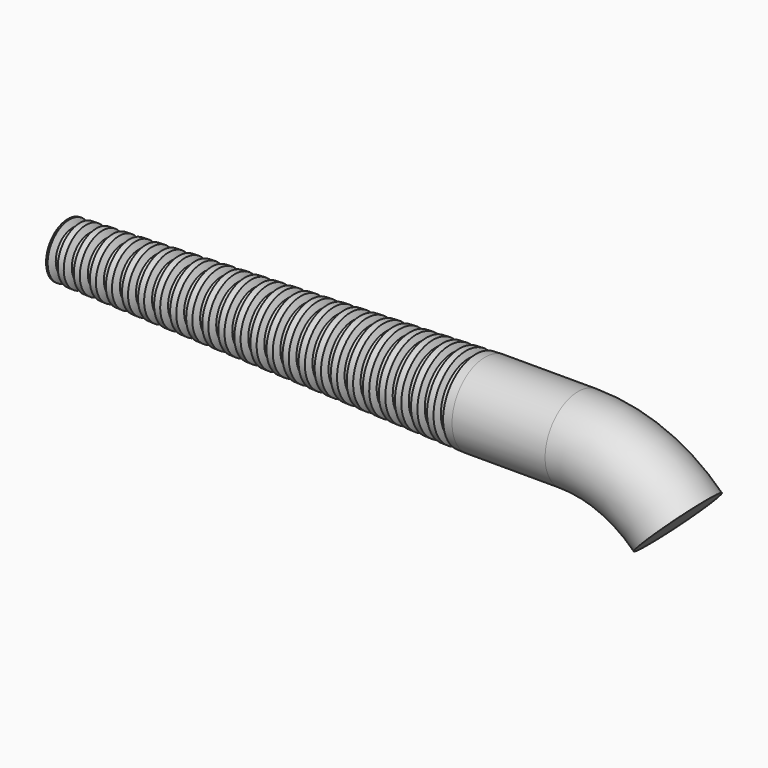
from build123d import *

# Parameters (mm, degrees)
F3_R      = 75
F8_R      = 49.537672475
F13_DEPTH = 232


with BuildPart() as f4:
    # F4: sweep along a path in F0
    with BuildLine(Plane.XZ) as f4_path:
        Line((-350, 75), (-181.066017178, 75))
        ThreePointArc((-181.066017178, 75), (0, 0), (75, -181.066017178))
        Line((75, -181.066017178), (75, -350))
    # F3 (on plane+point) → F4 (sweep)
    with BuildSketch(Plane.YZ.offset(-350)):
        with Locations((0, 75)):
            Circle(F3_R)
    sweep(path=f4_path.line)

    # F8 (on plane+point) → F9 section 0
    with BuildSketch(Plane.YZ.offset(-1107.697725296)):
        with Locations((0, 75)):
            Circle(F8_R)
    # F3 (on plane+point) → F9 section 1
    with BuildSketch(Plane.YZ.offset(-350)):
        with Locations((0, 75)):
            Circle(F3_R)
    loft()

    # F10 (on Front) → F11 (revolve, cut)
    with BuildSketch(Plane.XZ):
        Polygon((-1085.869221311, 125.2712163399), (-1104.697725296, 124.6384870611), (-1099.2664424752, 113.0726968058), (-1090.5117942881, 113.3668955503), align=None)
        Polygon((-1060.530301493, 114.4205035296), (-1055.8877285158, 126.3248243192), (-1074.7162325009, 125.6920950404), (-1069.28494968, 114.1263047851), align=None)
        Polygon((-1030.5488086978, 115.4741115089), (-1025.9062357207, 127.3784322985), (-1044.7347397057, 126.7457030197), (-1039.3034568849, 115.1799127644), align=None)
        Polygon((-1000.5673159027, 116.5277194882), (-995.9247429255, 128.4320402778), (-1014.7532469106, 127.799310999), (-1009.3219640897, 116.2335207437), align=None)
        Polygon((-970.5858231075, 117.5813274675), (-965.9432501303, 129.4856482571), (-984.7717541154, 128.8529189783), (-979.3404712946, 117.287128723), align=None)
        Polygon((-940.6043303123, 118.6349354468), (-935.9617573352, 130.5392562364), (-954.7902613202, 129.9065269576), (-949.3589784994, 118.3407367023), align=None)
        Polygon((-910.6228375172, 119.6885434262), (-905.98026454, 131.5928642158), (-924.8087685251, 130.960134937), (-919.3774857043, 119.3943446816), align=None)
        Polygon((-880.641344722, 120.7421514055), (-875.9987717449, 132.6464721951), (-894.8272757299, 132.0137429163), (-889.3959929091, 120.447952661), align=None)
        Polygon((-850.6598519269, 121.7957593848), (-846.0172789497, 133.7000801744), (-864.8457829348, 133.0673508956), (-859.4145001139, 121.5015606403), align=None)
        Polygon((-820.6783591317, 122.8493673641), (-816.0357861546, 134.7536881537), (-834.8642901396, 134.1209588749), (-829.4330073188, 122.5551686196), align=None)
        Polygon((-790.6968663366, 123.9029753434), (-786.0542933594, 135.807296133), (-804.8827973445, 135.1745668542), (-799.4515145236, 123.6087765989), align=None)
        Polygon((-760.7153735414, 124.9565833227), (-756.0728005643, 136.8609041123), (-774.9013045493, 136.2281748335), (-769.4700217285, 124.6623845782), align=None)
        Polygon((-730.7338807463, 126.010191302), (-726.0913077691, 137.9145120916), (-744.9198117542, 137.2817828128), (-739.4885289333, 125.7159925575), align=None)
        Polygon((-700.7523879511, 127.0637992813), (-696.1098149739, 138.9681200709), (-714.938318959, 138.3353907921), (-709.5070361382, 126.7696005368), align=None)
        Polygon((-670.770895156, 128.1174072606), (-666.1283221788, 140.0217280502), (-684.9568261639, 139.3889987714), (-679.525543343, 127.8232085161), align=None)
        Polygon((-640.7894023608, 129.17101524), (-636.1468293836, 141.0753360296), (-654.9753333687, 140.4426067508), (-649.5440505479, 128.8768164954), align=None)
        Polygon((-610.8079095656, 130.2246232193), (-606.1653365885, 142.1289440089), (-624.9938405735, 141.4962147301), (-619.5625577527, 129.9304244747), align=None)
        Polygon((-580.8264167705, 131.2782311986), (-576.1838437933, 143.1825519882), (-595.0123477784, 142.5498227094), (-589.5810649575, 130.9840324541), align=None)
        Polygon((-550.8449239753, 132.3318391779), (-546.2023509982, 144.2361599675), (-565.0308549832, 143.6034306887), (-559.5995721624, 132.0376404334), align=None)
        Polygon((-520.8634311802, 133.3854471572), (-516.220858203, 145.2897679468), (-535.0493621881, 144.657038668), (-529.6180793672, 133.0912484127), align=None)
        Polygon((-490.881938385, 134.4390551365), (-486.2393654079, 146.3433759261), (-505.0678693929, 145.7106466473), (-499.6365865721, 134.144856392), align=None)
        Polygon((-460.9004455899, 135.4926631158), (-456.2578726127, 147.3969839054), (-475.0863765978, 146.7642546266), (-469.6550937769, 135.1984643713), align=None)
        Polygon((-430.9189527947, 136.5462710951), (-426.2763798176, 148.4505918847), (-445.1048838026, 147.8178626059), (-439.6736009818, 136.2520723506), align=None)
        Polygon((-400.9374599996, 137.5998790744), (-396.2948870224, 149.504199864), (-415.1233910075, 148.8714705852), (-409.6921081866, 137.3056803299), align=None)
        Polygon((-370.9559672044, 138.6534870538), (-366.3133942272, 150.5578078433), (-385.1418982123, 149.9250785646), (-379.7106153915, 138.3592883092), align=None)
    revolve(axis=Axis((-609.0528770564, 0, 75), (-1, 0, 0)), mode=Mode.SUBTRACT)

    # F12 (on Front) → F13 (cut, symmetric)
    with BuildSketch(Plane.XZ):
        Polygon((98.1314237101, 98.1314237101), (-114.6691401448, -114.6691401448), (-121.5471847165, -389.7904326519), (441.9294075858, -378.4590830407), align=None)
    extrude(amount=F13_DEPTH, both=True, mode=Mode.SUBTRACT)


solid = f4.part
